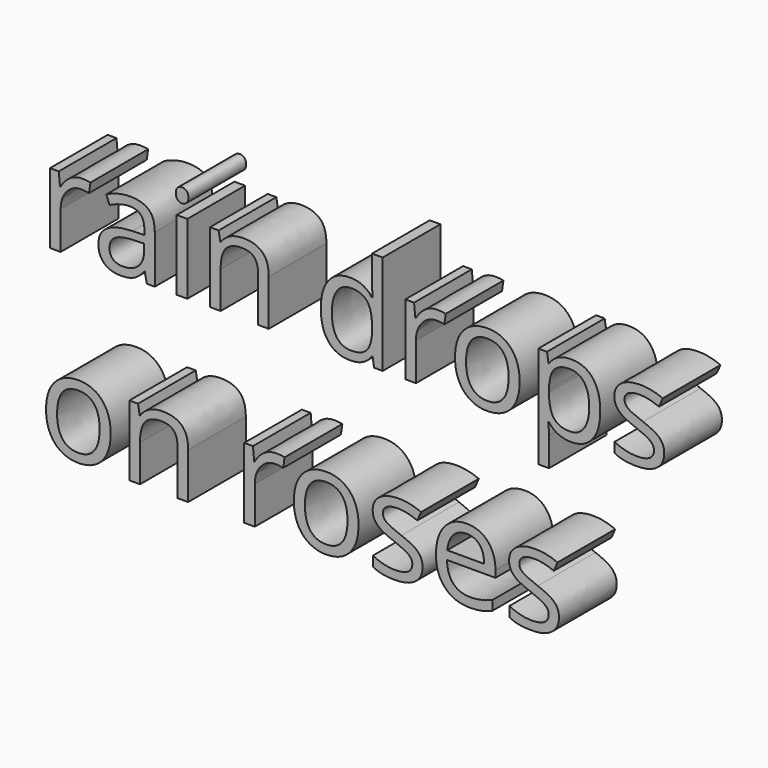
from build123d import *

# Parameters (mm, degrees)
F0_TEXT_SIZE = 46.283170943
F1_DEPTH     = 25.4


# Not quite as in the source:
# - Text() gives the source's letters only with a copy of the font that has no kerning and outlines rounded to 1/6400 em; it was checked with that copy


with BuildPart() as f1:
    # F0 (on Front) → F1 (new body)
    with BuildSketch(Plane.XZ):
        with Locations((-82.8944444656, -28.7172440439)):
            Text('rain drops', F0_TEXT_SIZE, font='Open Sans', text_align=(TextAlign.LEFT, TextAlign.BOTTOM))
        with Locations((-82.8944444656, -91.6623565265)):
            Text('on roses', F0_TEXT_SIZE, font='Open Sans', text_align=(TextAlign.LEFT, TextAlign.BOTTOM))
    extrude(amount=F1_DEPTH)


solid = f1.part
